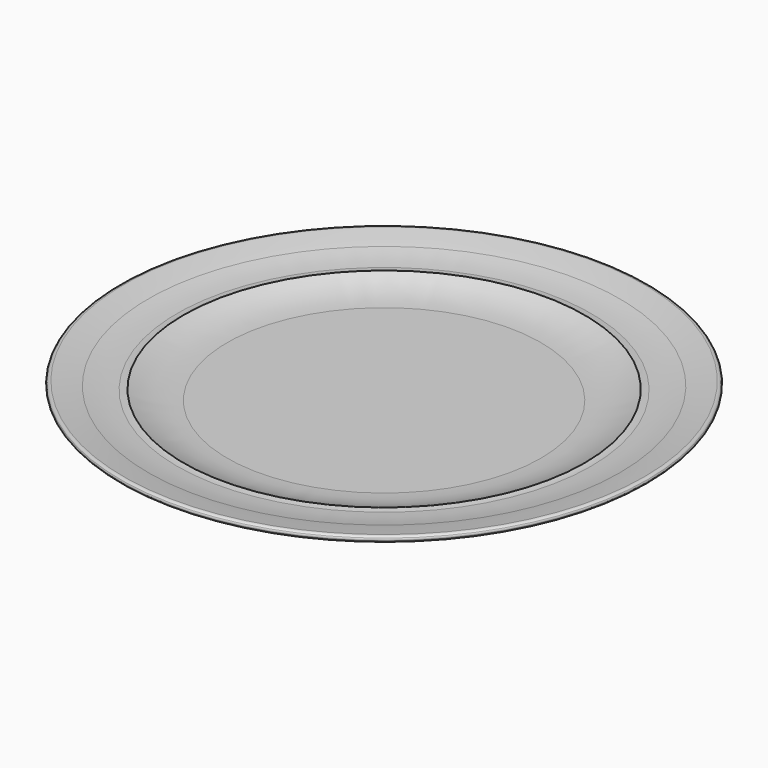
from build123d import *


# Not quite as in the source:
# - a fillet or chamfer that OpenCascade refuses, or shapes differently, is made with other operations: its cross-section is extruded or revolved along the edge and cut away or added


with BuildPart() as f1:
    # F0 (on Front) → F1 (revolve)
    with BuildSketch(Plane.XZ):
        with BuildLine():
            Line((100, 0), (0, 0))
            Line((0, 0), (0, -2.6495179627))
            Line((0, -2.6495179627), (91.3194956564, -2.6495179627))
            ThreePointArc((91.3194956564, -2.6495179627), (94.0684515249, -3.473007262), (95.9119130966, -5.6722213094))
            Line((95.9119130966, -5.6722213094), (95.9628000855, -5.7904100977))
            Line((95.9628000855, -5.7904100977), (98.6674576998, -5.7904100977))
            ThreePointArc((98.6674576998, -5.7904100977), (99.3204777078, -4.1476735329), (100.3251448274, -2.6931418106))
            ThreePointArc((100.3251448274, -2.6931418106), (101.5086125026, -1.71503666), (102.9425561428, -1.1663190089))
            ThreePointArc((102.9425561428, -1.1663190089), (109.6751369936, 0.1797320354), (116.4222210646, 1.4510914916))
            ThreePointArc((116.4222210646, 1.4510914916), (123.2251802907, 3.0758263676), (129.8146396875, 5.4208301008))
            ThreePointArc((129.8146396875, 5.4208301008), (130.7332526352, 5.961479711), (131.4723342657, 6.7295357585))
            ThreePointArc((131.4723342657, 6.7295357585), (131.6712873102, 7.3402645066), (131.4723342657, 7.9509932548))
            ThreePointArc((131.4723342657, 7.9509932548), (130.7405288737, 8.5304559761), (129.8146396875, 8.648969233))
            ThreePointArc((129.8146396875, 8.648969233), (123.6657142098, 7.6457790436), (117.5564303994, 6.4241709188))
            ThreePointArc((117.5564303994, 6.4241709188), (110.44281422, 5.2047996177), (103.2479256392, 4.6356073581))
            ThreePointArc((103.2479256392, 4.6356073581), (101.6107063419, 4.6996452731), (100, 5))
            Line((100, 5), (100, 0))
        make_face()
    revolve(axis=Axis((0, 0, -1.3247589814), (0, 0, -1)))

    # F2: fillet of radius 50 on 1 edges, made by hand

    # F2_s1 → F2_t2 (revolve)
    with BuildSketch(Plane.XZ):
        with BuildLine():
            ThreePointArc((100, 5), (89.3858451698, 1.266028276), (78.2055052823, 0))
            Line((78.2055052823, 0), (78.2055052823, -1))
            Line((78.2055052823, -1), (100, -1))
            Line((100, -1), (101, 0))
            ThreePointArc((101, 0), (101, 2.5), (100.4358898944, 4.1))
            Line((100.4358898944, 4.1), (100, 5))
        make_face()
    revolve(axis=Axis((0, 0, 0), (0, 0, -1)))


solid = f1.part
